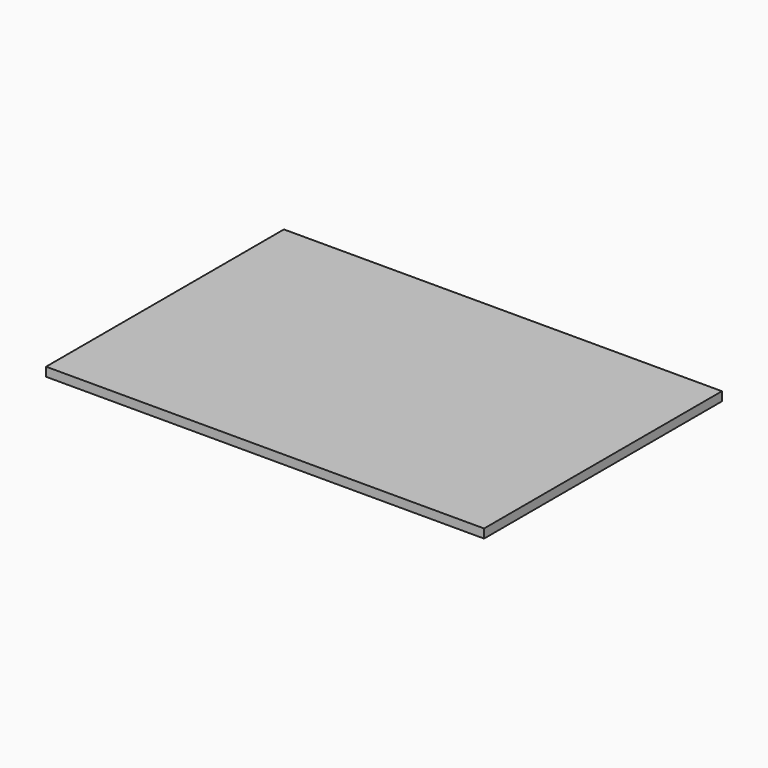
from build123d import *

# Parameters (mm, degrees)
F0_W     = 884
F0_H     = 600
F1_DEPTH = 18


# Not quite as in the source:
# - a feature of the source that left no trace in its solid (it failed there, or was rolled back) is left out


with BuildPart() as f1:
    # F0 (on Top) → F1 (new body)
    with BuildSketch(Plane.XY):
        with Locations((442, 300)):
            Rectangle(F0_W, F0_H)
    extrude(amount=F1_DEPTH)


solid = f1.part
